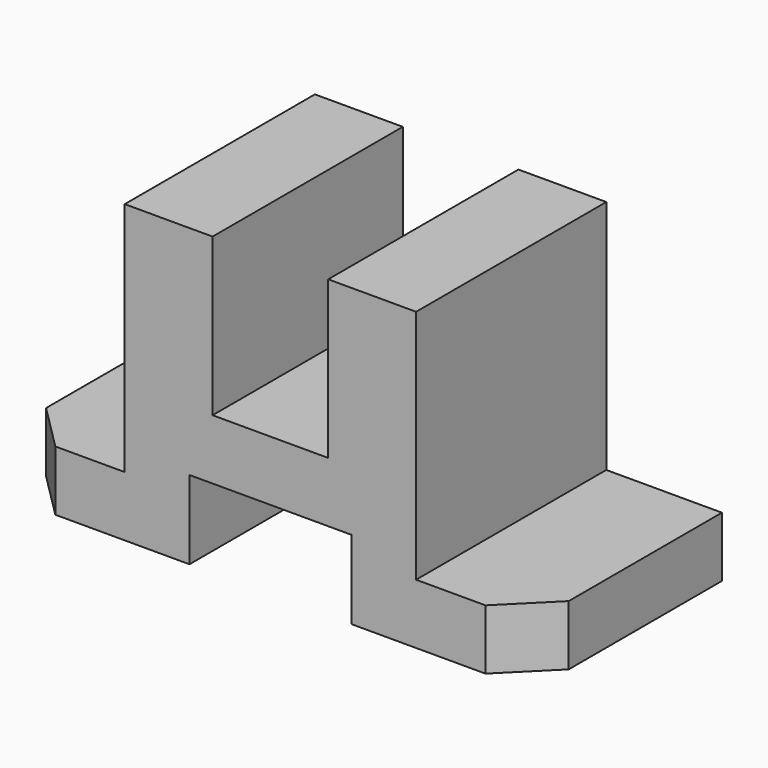
from build123d import *

# Parameters (mm, degrees)
F0_W      = 113
F0_H      = 26
F1_DEPTH  = 64
F2_W      = 25
F2_H      = 36.5019804899
F3_DEPTH  = 50.8
F4_W      = 25
F4_H      = 65.5092679775
F5_DEPTH  = 50.8
F6_DEPTH  = 25.4
F7_W      = 25
F7_H      = 54.8469666392
F8_DEPTH  = 50.8
F9_W      = 35
F9_H      = 17
F10_DEPTH = 50.8
F11_SIZE  = 10
F12_SIZE  = 10


# Not quite as in the source:
# - a feature of the source that left no trace in its solid (it failed there, or was rolled back) is left out


with BuildPart() as f1:
    # F0 (on Top) → F1 (new body)
    with BuildSketch(Plane.XY):
        with Locations((5.4938797247, 11.7718060501)):
            Rectangle(F0_W, F0_H)
    extrude(amount=F1_DEPTH)

    # F2 (on Front) → F3 (cut, symmetric)
    with BuildSketch(Plane.XZ):
        with Locations((5.4938797247, 48.2509902449)):
            Rectangle(F2_W, F2_H)
    extrude(amount=F3_DEPTH, both=True, mode=Mode.SUBTRACT)

    # F4 (on Front) → F5 (cut, symmetric)
    with BuildSketch(Plane.XZ):
        with Locations((-38.5061202753, 45.7546339888)):
            Rectangle(F4_W, F4_H)
    extrude(amount=F5_DEPTH, both=True, mode=Mode.SUBTRACT)

    # F6 (add): faces of the model
    f6_faces = [f1.faces().sort_by_distance(p)[0] for p in [
        (16.4788023799, -1.2281939499, 27.8806540043),
        (16.4788023799, 24.7718060501, 27.8806540043),
    ]]
    extrude(f6_faces, amount=F6_DEPTH, dir=(0, -1, 0))

    # F7 (on Front) → F8 (cut, symmetric)
    with BuildSketch(Plane.XZ):
        with Locations((49.4938797247, 40.4234833196)):
            Rectangle(F7_W, F7_H)
    extrude(amount=F8_DEPTH, both=True, mode=Mode.SUBTRACT)

    # F9 (on Front) → F10 (cut, symmetric)
    with BuildSketch(Plane.XZ):
        with Locations((5.4938797247, 8.5)):
            Rectangle(F9_W, F9_H)
    extrude(amount=F10_DEPTH, both=True, mode=Mode.SUBTRACT)

    # F11
    f11_edges = [f1.edges().sort_by_distance(p)[0] for p in [
        (61.99388, -26.628194, 6.5),
    ]]
    chamfer(f11_edges, length=F11_SIZE)

    # F12
    f12_edges = [f1.edges().sort_by_distance(p)[0] for p in [
        (-51.00612, -26.628194, 6.5),
    ]]
    chamfer(f12_edges, length=F12_SIZE)


solid = f1.part
